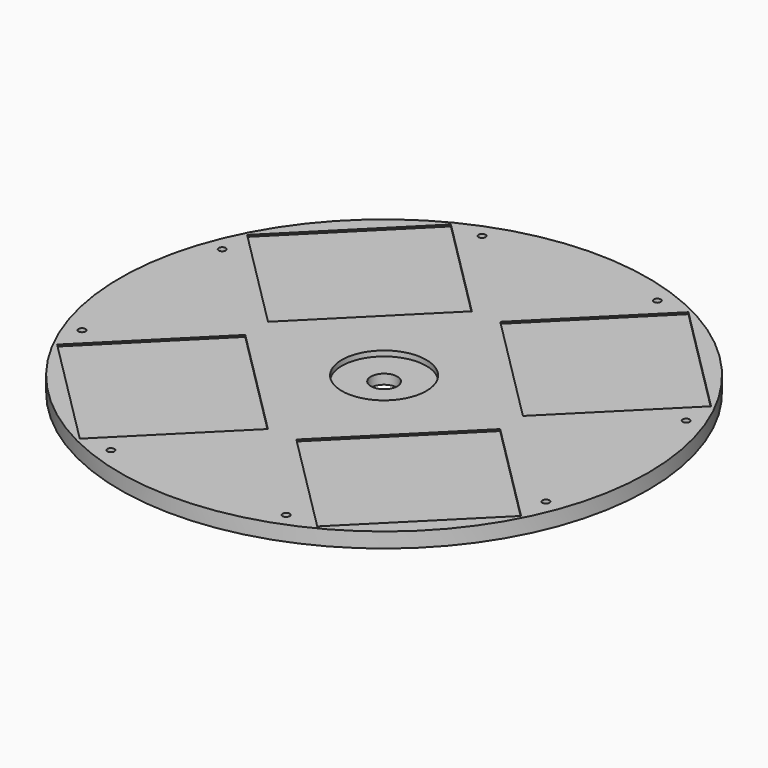
from build123d import *

# Parameters (mm, degrees)
F0_R     = 300
F1_DEPTH = 17.1
F3_DEPTH = 2
F4_R     = 4
F5_DEPTH = 25
F6_R     = 48
F7_DEPTH = 6
F8_R     = 15
F9_DEPTH = 11.101


# Not quite as in the source:
# - a feature names something its author has since deleted; it is built from what else it names


with BuildPart() as f1:
    # F0 (on Top) → F1 (new body)
    with BuildSketch(Plane.XY):
        Circle(F0_R)
    extrude(amount=F1_DEPTH)

    # F2 (on face) → F3 (cut)
    with BuildSketch(Plane.XY.offset(17.1)):
        Polygon((-144.8616802798, -16.1682461039), (-263.6556195192, -134.9621853432), (-134.9621853432, -263.6556195192), (-16.1682461039, -144.8616802798), align=None)
        Polygon((144.8616802798, -16.1682461039), (16.1682461039, -144.8616802798), (134.9621853432, -263.6556195192), (263.6556195192, -134.9621853432), align=None)
        Polygon((16.1682461039, 144.8616802798), (144.8616802798, 16.1682461039), (263.6556195192, 134.9621853432), (134.9621853432, 263.6556195192), align=None)
        Polygon((-144.8616802798, 16.1682461039), (-16.1682461039, 144.8616802798), (-134.9621853432, 263.6556195192), (-263.6556195192, 134.9621853432), align=None)
    extrude(amount=-F3_DEPTH, mode=Mode.SUBTRACT)

    # F4 (on face) → F5 (cut)
    with BuildSketch(Plane.XY.offset(17.1)):
        with Locations((-263.6556195192, -99.6068462839)):
            Circle(F4_R)
        with Locations((-99.6068462839, -263.6556195192)):
            Circle(F4_R)
        with Locations((99.6068462839, -263.6556195192)):
            Circle(F4_R)
        with Locations((263.6556195192, -99.6068462839)):
            Circle(F4_R)
        with Locations((263.6556195192, 99.6068462839)):
            Circle(F4_R)
        with Locations((99.6068462839, 263.6556195192)):
            Circle(F4_R)
        with Locations((-99.6068462839, 263.6556195192)):
            Circle(F4_R)
        with Locations((-263.6556195192, 99.6068462839)):
            Circle(F4_R)
    extrude(amount=-F5_DEPTH, mode=Mode.SUBTRACT)

    # F6 (on face) → F7 (cut)
    with BuildSketch(Plane.XY.offset(17.1)):
        Circle(F6_R)
    extrude(amount=-F7_DEPTH, mode=Mode.SUBTRACT)

    # F8 (on face) → F9 (cut, through all)
    with BuildSketch(Plane.XY.offset(11.1)):
        Circle(F8_R)
    extrude(amount=-F9_DEPTH, mode=Mode.SUBTRACT)


solid = f1.part
